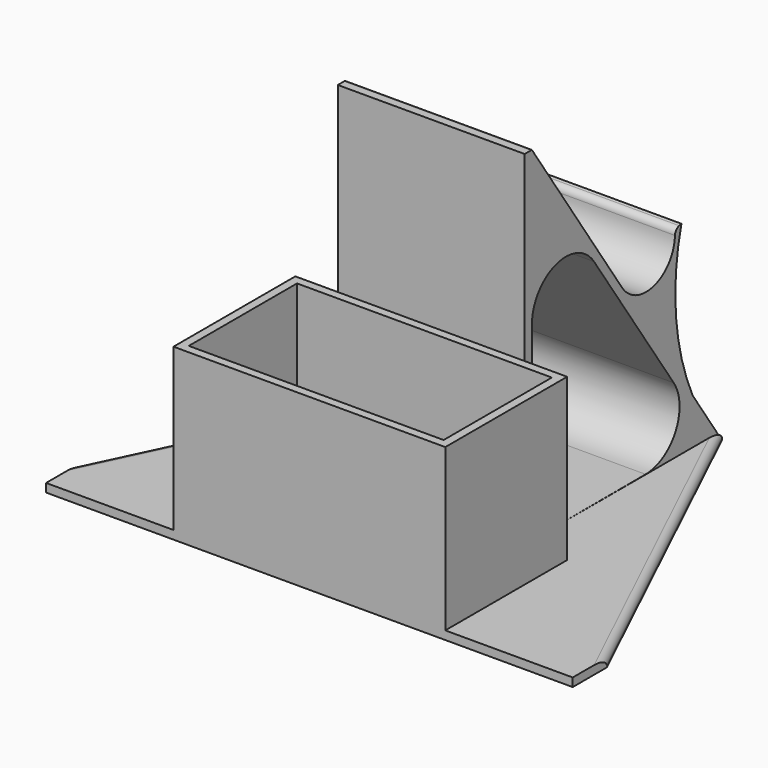
from build123d import *

# Parameters (mm, degrees)
F1_DEPTH     = 50.8
F0_W         = 27.7595084697
F0_H         = 50.8
F2_DEPTH     = 50.8
F3_DEPTH     = 5.08
F4_W         = 50.8
F4_H         = 22.6795084697
F5_DEPTH     = 48.26
F6_DEPTH     = 5.08
F7_DEPTH     = 5.08
F9_DEPTH     = 2.54
F10_DEPTH    = 2.54
F11_W        = 32.8395084697
F11_H        = 48.26
F12_DEPTH    = 12.7
F13_DEPTH    = 12.7
F14_DEPTH    = 12.7
F15_W        = 5.08
F15_H        = 48.26
F16_DEPTH    = 12.7
F17_DEPTH    = 12.7
F18_DEPTH    = 12.7
F19_DEPTH    = 12.7
F20_DEPTH    = 8.128
F21_T4_DEPTH = 128.2260634838
F21_T9_DEPTH = 128.2260634838
F22_DEPTH    = 55.88
F23_T1_DEPTH = 64.3167663813
F23_T3_DEPTH = 57.6244964954


# Not quite as in the source:
# - a fillet or chamfer that OpenCascade refuses, or shapes differently, is made with other operations: its cross-section is extruded or revolved along the edge and cut away or added


with BuildPart() as f1:
    # F0 (on Right) → F1 (new body)
    with BuildSketch(Plane.YZ):
        with BuildLine():
            Line((-71.0184, 0), (0, 0))
            Line((0, 0), (-10.9642549201, 16.2528208016))
            ThreePointArc((-10.9642549201, 16.2528208016), (-17.1471321538, 39.3310006748), (-15.1420671787, 63.1387740186))
            Line((-15.1420671787, 63.1387740186), (-17.6175407807, 62.569888753))
            ThreePointArc((-17.6175407807, 62.569888753), (-24.5875393509, 51.197400125), (-37.2879006076, 55.273575))
            Line((-37.2879006076, 55.273575), (-71.0245725858, 105.283))
            Line((-71.0245725858, 105.283), (-71.0245725858, 113.4411775106))
            Line((-71.0245725858, 113.4411775106), (-73.7388915303, 113.4411775106))
            Line((-73.7388915303, 113.4411775106), (-73.7388915303, 111.1043775106))
            Line((-73.7388915303, 111.1043775106), (-73.7388915303, 104.7543775106))
            Line((-73.7388915303, 104.7543775106), (-73.7388915303, 50.8))
            Line((-73.7388915303, 50.8), (-73.7388915303, 0))
            Line((-73.7388915303, 0), (-71.0184, 0))
        make_face()
        with BuildLine():
            Line((-71.0202538047, 15.2566983302), (-71.0245725858, 50.8))
            Line((-71.0245725858, 50.8), (-71.0245725858, 59.3205996023))
            ThreePointArc((-71.0245725858, 59.3205996023), (-62.0474659399, 71.4626778871), (-47.8072395033, 66.4392866182))
            Line((-47.8072395033, 66.4392866182), (-18.0124509852, 22.4196922368))
            ThreePointArc((-18.0124509852, 22.4196922368), (-17.3072850245, 9.3557957859), (-28.5115534391, 2.6010183058))
            Line((-28.5115534391, 2.6010183058), (-58.3020232698, 2.5582545615))
            ThreePointArc((-58.3020232698, 2.5582545615), (-67.2935162115, 6.2709969901), (-71.0202538047, 15.2566983302))
        make_face(mode=Mode.SUBTRACT)
    extrude(amount=F1_DEPTH)

    # F0 (on Right) → F2 (join)
    with BuildSketch(Plane.YZ):
        with Locations((-87.6186457652, 25.4)):
            Rectangle(F0_W, F0_H)
    extrude(amount=F2_DEPTH)

    # F3 (add): a face of the model
    f3_faces = [f1.faces().sort_by_distance(p)[0] for p in [
        (50.8, -72.5467692209, 109.3620887553),
    ]]
    extrude(f3_faces, amount=F3_DEPTH)

    # F4 (on face) → F5 (cut)
    with BuildSketch(Plane.XY.offset(50.8)):
        with Locations((27.94, -87.6186457652)):
            Rectangle(F4_W, F4_H)
    extrude(amount=-F5_DEPTH, mode=Mode.SUBTRACT)

    # F6 (add): a face of the model
    f6_faces = [f1.faces().sort_by_distance(p)[0] for p in [
        (27.94, -101.4984, 25.4),
    ]]
    extrude(f6_faces, amount=F6_DEPTH)

    # F7 (cut): a face of the model
    f7_faces = [f1.faces().sort_by_distance(p)[0] for p in [
        (27.94, -98.9584, 26.67),
    ]]
    extrude(f7_faces, amount=-F7_DEPTH, mode=Mode.SUBTRACT)

    # F8 (on face) → F9 (join)
    with BuildSketch(Plane(origin=(0, 0, 0), x_dir=(1, 0, 0), z_dir=(0, 0, -1))):
        Polygon((0, 0), (0, 106.5784), (-50.8, 106.5784), align=None)
    extrude(amount=-F9_DEPTH)

    # F8 (on face) → F10 (join)
    with BuildSketch(Plane(origin=(0, 0, 0), x_dir=(1, 0, 0), z_dir=(0, 0, -1))):
        Polygon((106.68, 106.5784), (55.88, 106.5784), (55.88, 0), align=None)
    extrude(amount=-F10_DEPTH)

    # F11 (on face) → F12 (join)
    with BuildSketch(Plane.YZ.offset(55.88)):
        with Locations((-90.1586457652, 26.67)):
            Rectangle(F11_W, F11_H)
    extrude(amount=F12_DEPTH)

    # F13 (cut): a face of the model
    f13_faces = [f1.faces().sort_by_distance(p)[0] for p in [
        (53.34, -90.1586457652, 26.67),
    ]]
    extrude(f13_faces, amount=-F13_DEPTH, mode=Mode.SUBTRACT)

    # F0 (on Right) → F14 (join)
    with BuildSketch(Plane.YZ):
        with Locations((-87.6186457652, 25.4)):
            Rectangle(F0_W, F0_H)
    extrude(amount=-F14_DEPTH)

    # F15 (on face) → F16 (join)
    with BuildSketch(Plane(origin=(0, 0, 0), x_dir=(0, -1, 0), z_dir=(-1, 0, 0))):
        with Locations((104.0384, 26.67)):
            Rectangle(F15_W, F15_H)
    extrude(amount=F16_DEPTH)

    # F17 (cut): a face of the model
    f17_faces = [f1.faces().sort_by_distance(p)[0] for p in [
        (2.54, -90.1586457652, 26.67),
    ]]
    extrude(f17_faces, amount=-F17_DEPTH, mode=Mode.SUBTRACT)

    # F18 (add): a face of the model
    f18_faces = [f1.faces().sort_by_distance(p)[0] for p in [
        (27.94, -106.5784, 24.3195522388),
    ]]
    extrude(f18_faces, amount=F18_DEPTH)

    # F19 (cut): a face of the model
    f19_faces = [f1.faces().sort_by_distance(p)[0] for p in [
        (27.94, -104.0384, 26.67),
    ]]
    extrude(f19_faces, amount=-F19_DEPTH, mode=Mode.SUBTRACT)

    # F20 (cut): a face of the model
    f20_faces = [f1.faces().sort_by_distance(p)[0] for p in [
        (27.94, -72.3817320581, 113.4411775106),
    ]]
    extrude(f20_faces, amount=-F20_DEPTH, mode=Mode.SUBTRACT)

    # F21: fillet of radius 2.032 on 2 edges, made by hand


with BuildPart() as f21_tool2:
    # F21_s3 → F21_t4 (new body)
    with BuildSketch(Plane(origin=(8.1593159461, -17.1182448549, 0), x_dir=(0, 0, 1), z_dir=(0.430267585, -0.9027013932, 0))):
        with BuildLine():
            ThreePointArc((2.54, -48.4109538537), (1.9448409794, -49.8477948331), (0.508, -50.4429538537))
            Line((0.508, -50.4429538537), (2.54, -50.4429538537))
            Line((2.54, -50.4429538537), (2.54, -48.4109538537))
        make_face()
    extrude(amount=F21_T4_DEPTH)

    split(bisect_by=Plane.YZ.offset(55.88), keep=Keep.TOP)


with BuildPart() as f1_1:
    add(f1.part)

    # F21_t1: cut F21_tool2
    add(f21_tool2.part, mode=Mode.SUBTRACT)


with BuildPart() as f21_tool7:
    # F21_s8 → F21_t9 (new body)
    with BuildSketch(Plane(origin=(-52.9857593316, -111.1641230776, 0), x_dir=(0, 0, 1), z_dir=(0.430267585, 0.9027013932, 0))):
        with BuildLine():
            ThreePointArc((2.54, 2.032), (1.9448409794, 0.5951590206), (0.508, 0))
            Line((0.508, 0), (2.54, 0))
            Line((2.54, 0), (2.54, 2.032))
        make_face()
    extrude(amount=F21_T9_DEPTH)

    split(bisect_by=Plane.YZ, keep=Keep.BOTTOM)


with BuildPart() as f1_2:
    add(f1_1.part)

    # F21_t6: cut F21_tool7
    add(f21_tool7.part, mode=Mode.SUBTRACT)

    # F22 (add): a face of the model
    f22_faces = [f1_2.faces().sort_by_distance(p)[0] for p in [
        (55.88, -0.4726159714, 1.0164297188),
    ]]
    extrude(f22_faces, amount=F22_DEPTH)

    # F23: fillet of radius 2.032 on 2 edges, made by hand

    # F23_s2 → F23_t1 (cut)
    with BuildSketch(Plane.YZ.offset(-4.2183831906)):
        with BuildLine():
            ThreePointArc((-17.5491731756, 61.0234272483), (-17.0899741767, 62.2549630593), (-15.9730531852, 62.9478062399))
            Line((-15.9730531852, 62.9478062399), (-17.6175407807, 62.569888753))
            ThreePointArc((-17.6175407807, 62.569888753), (-17.5556082132, 61.7978847474), (-17.5491731756, 61.0234272483))
        make_face()
    extrude(amount=F23_T1_DEPTH, mode=Mode.SUBTRACT)

    # F23_s4 → F23_t3 (cut)
    with BuildSketch(Plane.YZ.offset(-0.8722482477)):
        with BuildLine():
            ThreePointArc((-71.0245725858, 105.283), (-71.1983709119, 105.3056190754), (-71.3734718849, 105.3131775106))
            Line((-71.3734718849, 105.3131775106), (-71.0245725858, 105.3131775106))
            Line((-71.0245725858, 105.3131775106), (-71.0245725858, 105.283))
        make_face()
    extrude(amount=F23_T3_DEPTH, mode=Mode.SUBTRACT)


solid = f1_2.part
